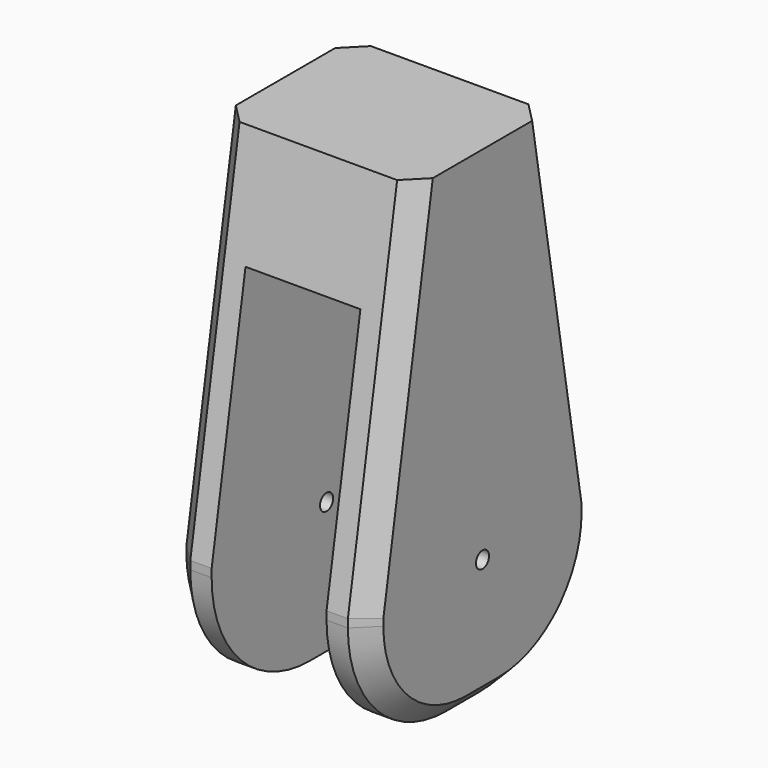
from build123d import *

# Parameters (mm, degrees)
F0_R     = 5
F1_DEPTH = 60
F3_W     = 226.6252040863
F3_H     = 197.2780163714
F3_H_2   = 59.4672214857
F4_DEPTH = 35
F5_R     = 75
F6_SIZE  = 12


# Not quite as in the source:
# - a feature names something its author has since deleted; it is built from what else it names


with BuildPart() as f1:
    # F0 (on Right) → F1 (new body, symmetric)
    with BuildSketch(Plane.YZ):
        Polygon((-87.5, -90), (-87.5, -170), (87.5, -170), (87.5, -90), (50, 130), (-50, 130), align=None)
        with Locations((0, -90)):
            Circle(F0_R, mode=Mode.SUBTRACT)
    extrude(amount=F1_DEPTH, both=True)

    # F3 (on face) → F4 (cut, symmetric)
    with BuildSketch(Plane.YZ):
        with Locations((-5.2212774754, -37.3711218749)):
            Rectangle(F3_W, F3_H)
        with Locations((-5.2212774754, -165.7437408035)):
            Rectangle(F3_W, F3_H_2)
    extrude(amount=F4_DEPTH, both=True, mode=Mode.SUBTRACT)

    # F5
    f5_edges = [f1.edges().sort_by_distance(p)[0] for p in [
        (-47.5, 87.5, -170),
        (47.5, 87.5, -170),
        (47.5, -87.5, -170),
        (-47.5, -87.5, -170),
    ]]
    fillet(f5_edges, radius=F5_R)

    # F6
    f6_edges = [f1.edges().sort_by_distance(p)[0] for p in [
        (60, 68.75, 20),
        (-60, 68.75, 20),
        (60, -65.533009, -148.033009),
        (60, -68.75, 20),
        (-60, -65.533009, -148.033009),
        (-60, -68.75, 20),
    ]]
    chamfer(f6_edges, length=F6_SIZE)


solid = f1.part
